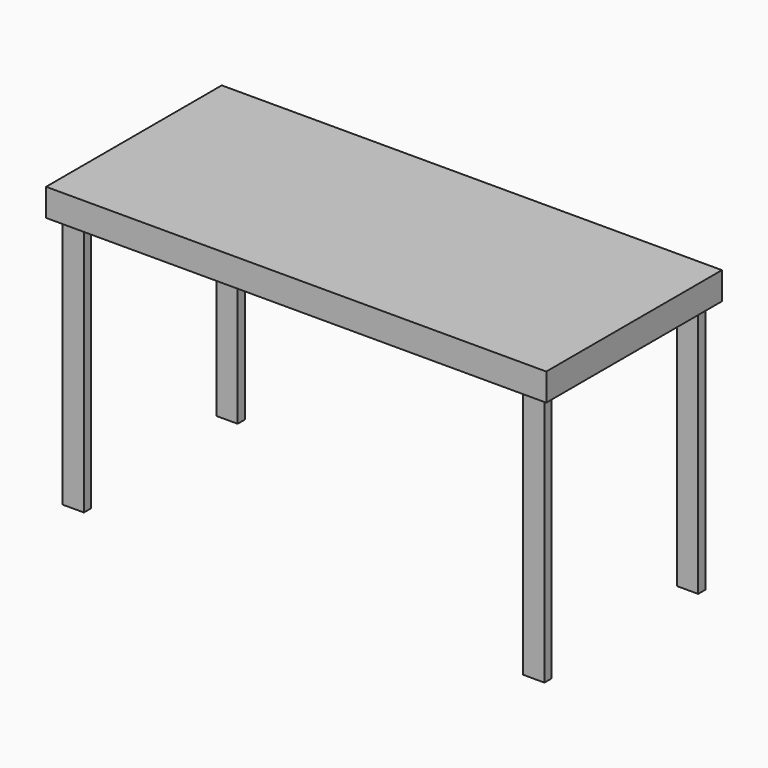
from build123d import *

# Parameters (mm, degrees)
F0_W     = 2082.8
F0_H     = 914.4
F1_DEPTH = 25.4
F2_W     = 38.1
F2_H     = 88.9
F3_DEPTH = 2082.8
F4_W     = 38.1
F4_H     = 88.9
F5_DEPTH = 838.2
F6_W     = 88.9
F6_H     = 38.1
F7_DEPTH = 1143


# Not quite as in the source:
# - a feature names something its author has since deleted; it is built from what else it names


with BuildPart() as f1:
    # F0 (on Top) → F1 (new body)
    with BuildSketch(Plane.XY):
        with Locations((1041.4, -457.2)):
            Rectangle(F0_W, F0_H)
    extrude(amount=F1_DEPTH)

    # F2 (on face) → F3 (join, through all)
    with BuildSketch(Plane.YZ.offset(2082.8)):
        with Locations((-895.35, -44.45)):
            Rectangle(F2_W, F2_H)
        with Locations((-19.05, -44.45)):
            Rectangle(F2_W, F2_H)
    extrude(amount=-F3_DEPTH)

    # F4 (on face) → F5 (join, through all)
    with BuildSketch(Plane.XZ.offset(38.1)):
        with Locations((19.05, -44.45)):
            Rectangle(F4_W, F4_H)
        with Locations((2063.75, -44.45)):
            Rectangle(F4_W, F4_H)
    extrude(amount=F5_DEPTH)

    # F6 (on face) → F7 (join)
    with BuildSketch(Plane(origin=(0, 0, 0), x_dir=(1, 0, 0), z_dir=(0, 0, -1))):
        with Locations((82.55, 857.25)):
            Rectangle(F6_W, F6_H)
        with Locations((82.55, 57.15)):
            Rectangle(F6_W, F6_H)
        with Locations((2000.25, 57.15)):
            Rectangle(F6_W, F6_H)
        with Locations((2000.25, 857.25)):
            Rectangle(F6_W, F6_H)
    extrude(amount=F7_DEPTH)


solid = f1.part
